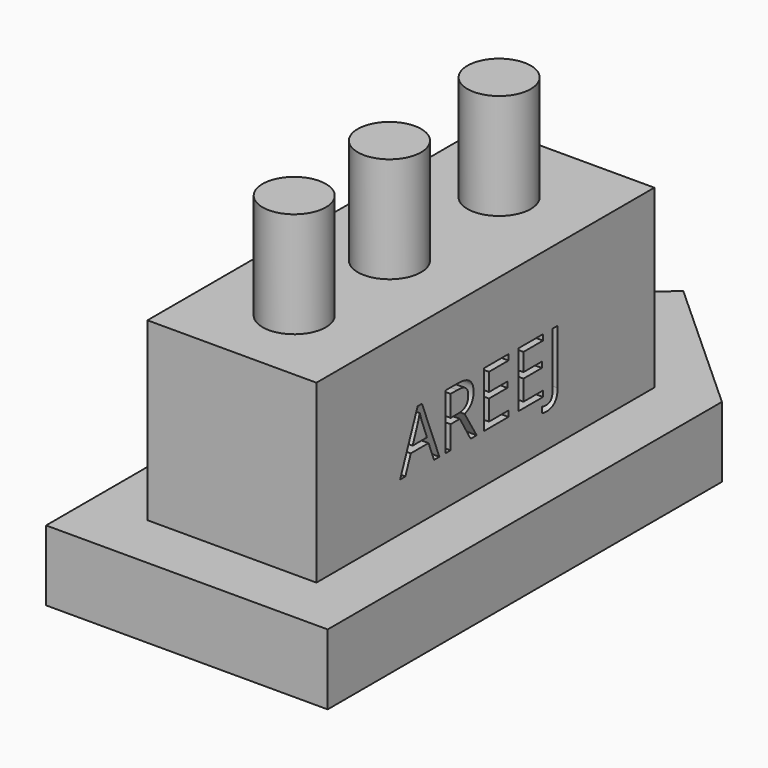
from build123d import *

# Parameters (mm, degrees)
F1_DEPTH     = 10
F2_W         = 24
F2_H         = 60
F3_DEPTH     = 25
F4_R         = 4.5
F5_DEPTH     = 15
F7_TEXT_SIZE = 11.0161878789
F8_DEPTH     = 5
F6_TEXT_SIZE = 10.2293134357
F9_DEPTH     = 5


# Not quite as in the source:
# - Text() gives the source's letters only with a copy of the font that has no kerning and outlines rounded to 1/6400 em; it was checked with that copy


with BuildPart() as f1:
    # F0 (on Top) → F1 (new body)
    with BuildSketch(Plane.XY):
        Polygon((-19.999999553, -40.5686236918), (20.000000447, -40.5686236918), (20.000000447, 29.4313763082), (4.47e-07, 47.5697334554), (-19.999999553, 29.4313763082), align=None)
    extrude(amount=F1_DEPTH)

    # F2 (on face) → F3 (join)
    with BuildSketch(Plane.XY.offset(10)):
        with Locations((4.47e-07, -2.5686236918)):
            Rectangle(F2_W, F2_H)
    extrude(amount=F3_DEPTH)

    # F4 (on face) → F5 (join)
    with BuildSketch(Plane.XY.offset(35)):
        with Locations((0, 14.8718534037)):
            Circle(F4_R)
        with Locations((0, -4.5979236992)):
            Circle(F4_R)
        with Locations((0, -21.5101772033)):
            Circle(F4_R)
    extrude(amount=F5_DEPTH)

    # F7 (on face) → F8 (cut)
    with BuildSketch(Plane.YZ.offset(12.000000447)):
        with Locations((-17.7045885939, 16.8547667563)):
            Text('AREEJ', F7_TEXT_SIZE, font='Open Sans', text_align=(TextAlign.LEFT, TextAlign.BOTTOM))
    extrude(amount=-F8_DEPTH, mode=Mode.SUBTRACT)

    # F6 (on face) → F9 (cut)
    with BuildSketch(Plane(origin=(-11.999999553, 0, 0), x_dir=(0, -1, 0), z_dir=(-1, 0, 0))):
        with Locations((-11.1892959103, 17.7045892924)):
            Text('LAMA', F6_TEXT_SIZE, font='Open Sans', text_align=(TextAlign.LEFT, TextAlign.BOTTOM))
    extrude(amount=-F9_DEPTH, mode=Mode.SUBTRACT)


solid = f1.part
